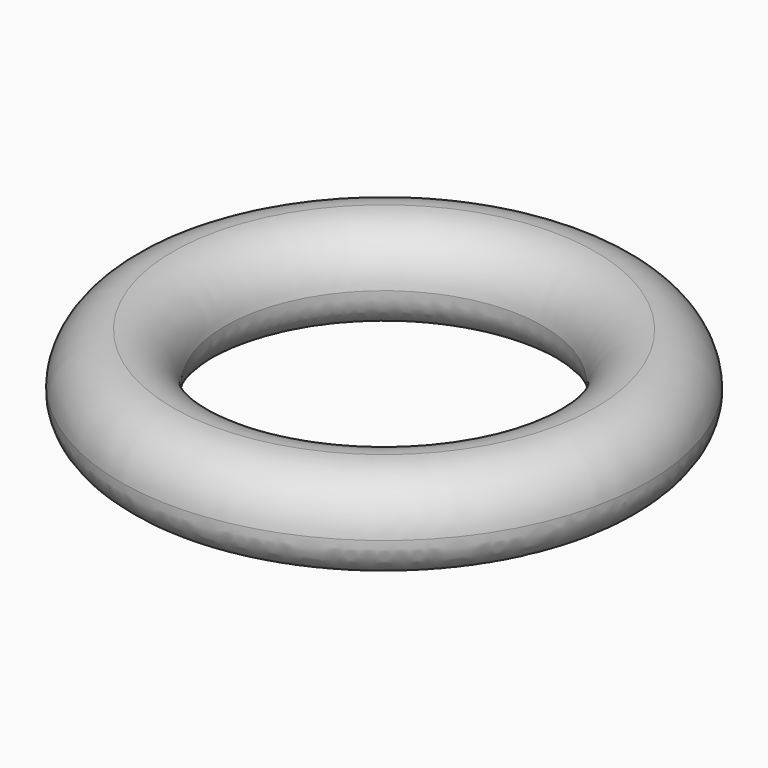
from build123d import *

# Parameters (mm, degrees)
F0_R     = 5
F0_R_2   = 3
F1_DEPTH = 1.7
F2_R     = 0.99999
F3_R     = 0.7242640687


# Not quite as in the source:
# - a fillet or chamfer is up to 0.001 mm smaller than in the source, because OpenCascade refuses the exact size


with BuildPart() as f1:
    # F0 (on Top) → F1 (new body)
    with BuildSketch(Plane.XY):
        Circle(F0_R)
        Circle(F0_R_2, mode=Mode.SUBTRACT)
    extrude(amount=F1_DEPTH)

    # F2 (radius 1 in the source; OpenCascade refuses exactly that, so slightly less here)
    f2_edges = [f1.edges().sort_by_distance(p)[0] for p in [
        (-5, 0, 1.7),
        (-3, 0, 1.7),
    ]]
    fillet(f2_edges, radius=F2_R)

    # F3
    f3_edges = [f1.edges().sort_by_distance(p)[0] for p in [
        (-5, 0, 0),
        (-3, 0, 0),
    ]]
    fillet(f3_edges, radius=F3_R)


solid = f1.part
